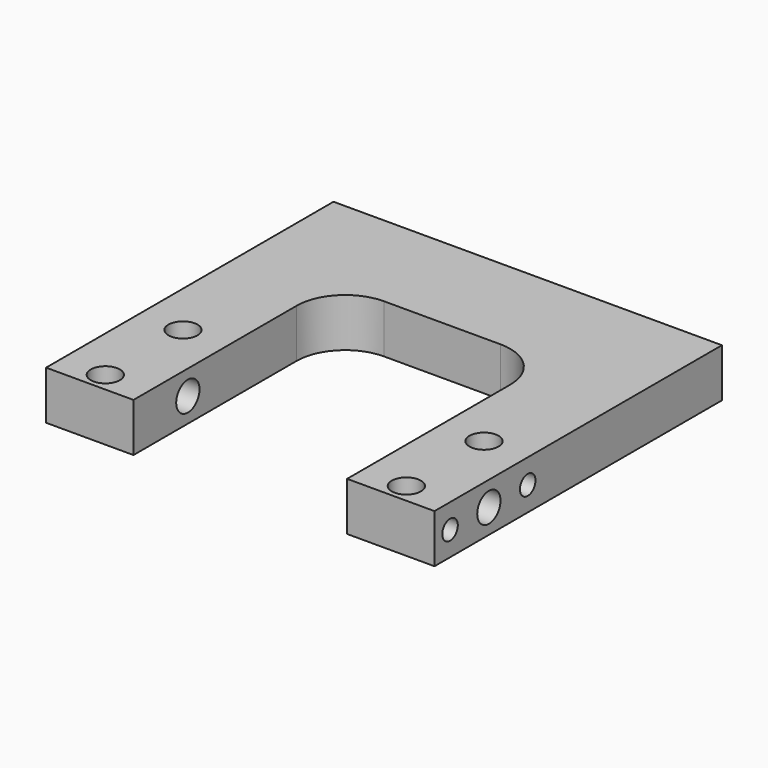
from build123d import *

# Parameters (mm, degrees)
F0_R     = 1.5
F1_DEPTH = 5
F3_D     = 2
F3_DEPTH = 5
F3_TIP   = 0.600860619
F4_R     = 5
F5_D     = 3


# Not quite as in the source:
# - a feature names something its author has since deleted; it is built from what else it names


with BuildPart() as f1:
    # F0 (on Top) → F1 (new body)
    with BuildSketch(Plane.XY):
        Polygon((11, 33), (11, 7), (20, 7), (20, 44), (0, 44), (0, 33), align=None)
        with Locations((15.5, 9)):
            Circle(F0_R, mode=Mode.SUBTRACT)
        with Locations((15.5, 19)):
            Circle(F0_R, mode=Mode.SUBTRACT)
    extrude(amount=-F1_DEPTH)

    # F3
    with Locations(Plane.YZ.offset(20)):
        with Locations((9, -2.5), (19, -2.5)):
            Hole(F3_D / 2, depth=F3_DEPTH)
            with Locations((0, 0, -(F3_DEPTH + F3_TIP / 2))):  # 118° drill point
                Cone(0, F3_D / 2, F3_TIP, mode=Mode.SUBTRACT)

    # F4
    f4_edges = [f1.edges().sort_by_distance(p)[0] for p in [
        (11, 33, -2.5),
    ]]
    fillet(f4_edges, radius=F4_R)

    # F5 (through all)
    with Locations(Plane.YZ.offset(20)):
        with Locations((14, -2.5)):
            Hole(F5_D / 2)

    # F6: F1 across plane


with BuildPart() as f1_1:
    add(f1.part)
    add(f1.part.mirror(Plane.YZ))


solid = f1_1.part
